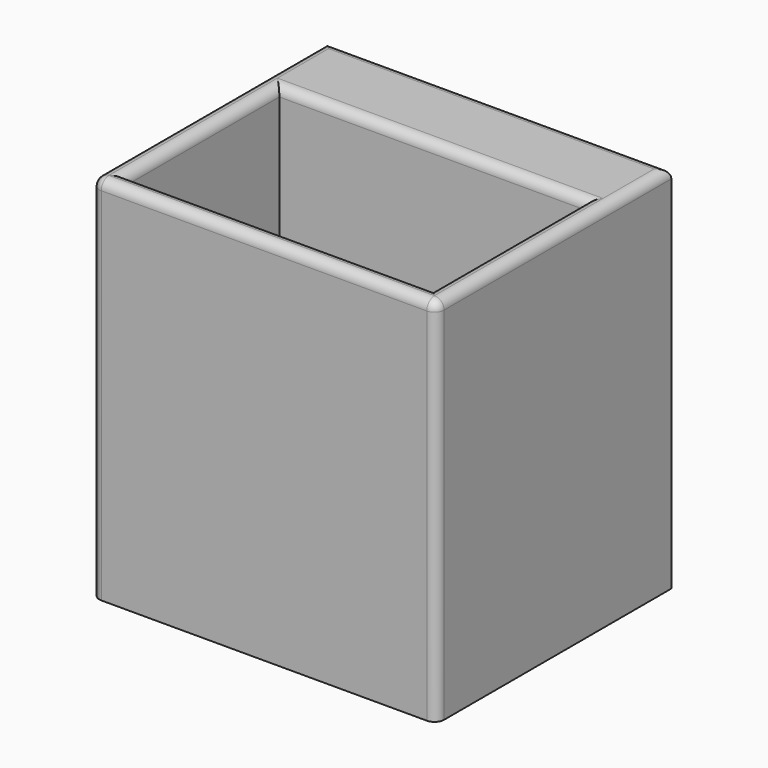
from build123d import *

# Parameters (mm, degrees)
F0_W     = 54
F0_H     = 36
F1_DEPTH = 58
F2_T     = -3
F3_W     = 54
F3_H     = 58
F4_DEPTH = 10
F5_R     = 1.49999


# Not quite as in the source:
# - a fillet or chamfer is up to 0.001 mm smaller than in the source, because OpenCascade refuses the exact size


with BuildPart() as f1:
    # F0 (on Top) → F1 (new body)
    with BuildSketch(Plane.XY):
        Rectangle(F0_W, F0_H)
    extrude(amount=F1_DEPTH)

    # F2
    f2_openings = [f1.faces().sort_by_distance(p)[0] for p in [
        (0, 0, 58),
    ]]
    offset(amount=F2_T, openings=f2_openings)

    # F3 (on face) → F4 (join)
    with BuildSketch(Plane(origin=(0, 18, 0), x_dir=(-1, 0, 0), z_dir=(0, 1, 0))):
        with Locations((0, 29)):
            Rectangle(F3_W, F3_H)
    extrude(amount=F4_DEPTH)

    # F5 (radius 1.5 in the source; OpenCascade refuses exactly that, so slightly less here)
    f5_edges = [f1.edges().sort_by_distance(p)[0] for p in [
        (0, -18, 58),
        (27, 5, 58),
        (0, 28, 58),
        (-27, 5, 58),
        (0, -15, 58),
        (-24, 0, 58),
        (0, 15, 58),
        (24, 0, 58),
        (-27, -18, 29),
        (27, -18, 29),
    ]]
    fillet(f5_edges, radius=F5_R)


solid = f1.part
